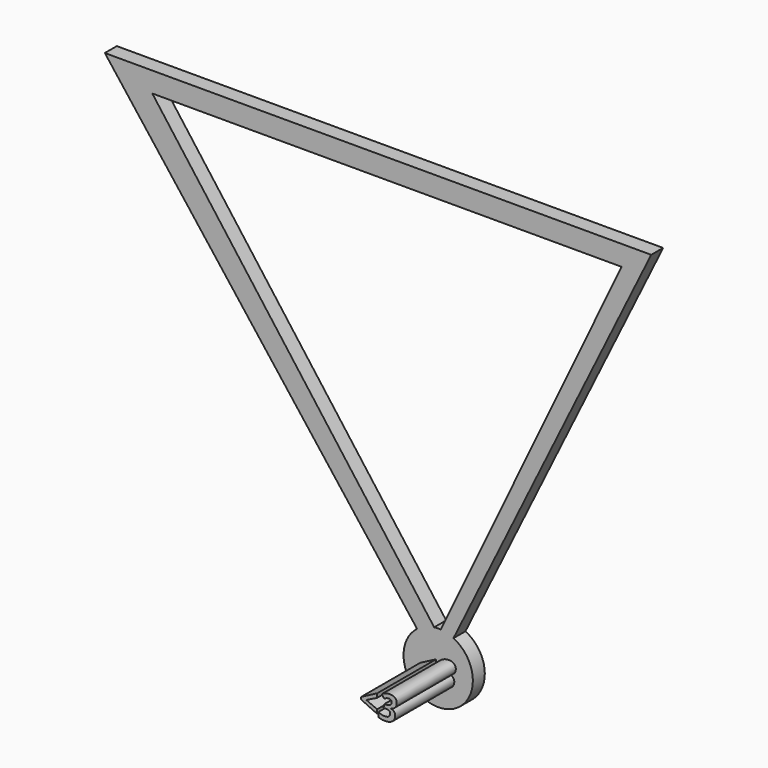
from build123d import *

# Parameters (mm, degrees)
F1_DEPTH     = 4.21
F2_R         = 9.7597636562
F3_DEPTH     = 4.21
F4_TEXT_SIZE = 9.6623061432
F5_DEPTH     = 25


# Not quite as in the source:
# - Text() gives the source's letters only with a copy of the font that has no kerning and outlines rounded to 1/6400 em; it was checked with that copy


with BuildPart() as f1:
    # F0 (on Front) → F1 (new body)
    with BuildSketch(Plane.XZ):
        Polygon((59.9878368103, 47.3457782139), (-93.8821631897, 47.3457782139), (0, -74.5645016432), align=None)
        Polygon((0, -66.3799643517), (-80.5216282606, 41.6559316218), (51.6586452723, 41.6559316218), align=None, mode=Mode.SUBTRACT)
    extrude(amount=F1_DEPTH)

    # F2 (on Front) → F3 (join)
    with BuildSketch(Plane.XZ):
        with Locations((0, -74.5645016432)):
            Circle(F2_R)
    extrude(amount=F3_DEPTH)

    # F4 (on Front) → F5 (join)
    with BuildSketch(Plane.XZ):
        with Locations((-5.5753849447, -78.6567516625)):
            Text('<3', F4_TEXT_SIZE, font='Open Sans', font_style=FontStyle.BOLDITALIC, text_align=(TextAlign.LEFT, TextAlign.BOTTOM))
    extrude(amount=F5_DEPTH)


solid = f1.part
